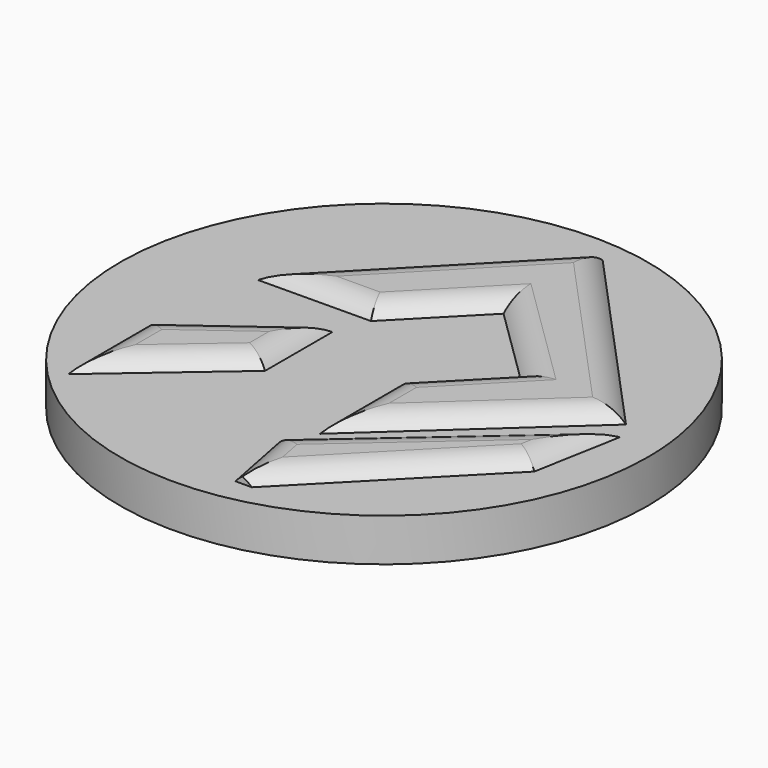
from build123d import *

# Parameters (mm, degrees)
F1_R         = 43.0886477689
F2_DEPTH     = 7
F3_DEPTH     = 9
F4_T1_DEPTH  = 65.4537906692
F4_T3_DEPTH  = 64.2896699852
F4_T5_DEPTH  = 38.3423168452
F4_T7_DEPTH  = 27.0257675551
F4_T9_DEPTH  = 18.685309
F4_T11_DEPTH = 25.5512004517
F4_T13_DEPTH = 59.0901082548
F4_T15_DEPTH = 43.6259466426
F4_T17_DEPTH = 36.1199672148
F4_T19_DEPTH = 45.1090392988
F4_T21_DEPTH = 31.581321794
F4_T23_DEPTH = 56.2861348222
F4_T25_DEPTH = 34.5042209979
F4_T27_DEPTH = 63.7210704382
F4_T32_DEPTH = 36.3207046716
F4_T37_DEPTH = 33.7416105717
F4_T43_DEPTH = 37.0257675551
F4_T47_DEPTH = 28.685309
F4_T54_DEPTH = 28.685309
F4_T58_DEPTH = 35.5512004517


# Not quite as in the source:
# - a fillet or chamfer that OpenCascade refuses, or shapes differently, is made with other operations: its cross-section is extruded or revolved along the edge and cut away or added


with BuildPart() as f2:
    # F1 (on Top) → F2 (new body)
    with BuildSketch(Plane.XY):
        with Locations((0, 9.9098170176)):
            Circle(F1_R)
    extrude(amount=F2_DEPTH)

    # F0 (on Top) → F3 (join)
    with BuildSketch(Plane.XY):
        Polygon((4.6245767735, 48.7562939525), (-26.2940470129, 17.0448832214), (-7.9522941785, 17.1887241356), (3.9733163334, 29.3401263082), (17.3091441393, 16.252098605), (6.4163865013, 5.1531046629), (6.4163865013, -11.1676000087), (35.278942436, 15.1950521395), align=None)
        Polygon((-9.9098188803, 11.7596480995), (-28.9366655052, -2.2462243214), (-28.9366655052, -18.3661915362), (-9.9098188803, -1.9819624722), align=None)
        Polygon((6.2101469375, -28.1438771635), (8.8527640328, -28.1438771635), (34.2691988262, -2.2462243214), (36.864515394, 12.0239108801), (3.9733163334, -16.7806204408), align=None)
    extrude(amount=F3_DEPTH)

    # F4: fillet of radius 5 on 17 edges, made by hand

    # F4_s2 → F4_t1 (cut)
    with BuildSketch(Plane(origin=(15.2233690689, -16.6669627471, 0), x_dir=(0, 0, 1), z_dir=(-0.6744072433, 0.7383595806, 0))):
        with BuildLine():
            ThreePointArc((7, 36.2961983644), (8.472135955, 34.5322663419), (9, 32.2961983644))
            Line((9, 32.2961983644), (9, 36.2961983644))
            Line((9, 36.2961983644), (7, 36.2961983644))
        make_face()
    extrude(amount=F4_T1_DEPTH, mode=Mode.SUBTRACT)

    # F4_s4 → F4_t3 (cut)
    with BuildSketch(Plane(origin=(33.6050957981, 34.4667667899, 0), x_dir=(0, 0, 1), z_dir=(-0.6981001167, -0.7160001585, 0))):
        with BuildLine():
            ThreePointArc((7, 30.7255767963), (8.472135955, 28.9616447738), (9, 26.7255767963))
            Line((9, 26.7255767963), (9, 30.7255767963))
            Line((9, 30.7255767963), (7, 30.7255767963))
        make_face()
    extrude(amount=F4_T3_DEPTH, mode=Mode.SUBTRACT)

    # F4_s6 → F4_t5 (cut)
    with BuildSketch(Plane(origin=(-36.1584602101, -0.2835642821, 0), x_dir=(0, 0, 1), z_dir=(0.9999692508, 0.0078420254, 0))):
        with BuildLine():
            ThreePointArc((7, -17.2505576897), (8.472135955, -19.0144897122), (9, -21.2505576897))
            Line((9, -21.2505576897), (9, -17.2505576897))
            Line((9, -17.2505576897), (7, -17.2505576897))
        make_face()
    extrude(amount=F4_T5_DEPTH, mode=Mode.SUBTRACT)

    # F4_s8 → F4_t7 (cut)
    with BuildSketch(Plane(origin=(-2.3131754341, -2.3569715754, 0), x_dir=(0, 0, 1), z_dir=(0.7004448095, 0.7137065705, 0))):
        with BuildLine():
            ThreePointArc((7, -17.7153572089), (8.472135955, -19.4792892314), (9, -21.7153572089))
            Line((9, -21.7153572089), (9, -17.7153572089))
            Line((9, -17.7153572089), (7, -17.7153572089))
        make_face()
    extrude(amount=F4_T7_DEPTH, mode=Mode.SUBTRACT)

    # F4_s10 → F4_t9 (cut)
    with BuildSketch(Plane(origin=(-12.6435668395, 12.4086300056, 0), x_dir=(0, 0, 1), z_dir=(0.7137065705, -0.7004448095, 0))):
        with BuildLine():
            ThreePointArc((7, -23.7233297289), (8.472135955, -25.4872617514), (9, -27.7233297289))
            Line((9, -27.7233297289), (9, -23.7233297289))
            Line((9, -23.7233297289), (7, -23.7233297289))
        make_face()
    extrude(amount=F4_T9_DEPTH, mode=Mode.SUBTRACT)

    # F4_s12 → F4_t11 (cut)
    with BuildSketch(Plane(origin=(16.6168831729, 16.9314963026, 0), x_dir=(0, 0, 1), z_dir=(-0.7004448095, -0.7137065705, 0))):
        with BuildLine():
            ThreePointArc((7, -0.9699517911), (8.472135955, -2.7338838136), (9, -4.9699517911))
            Line((9, -4.9699517911), (9, -0.9699517911))
            Line((9, -0.9699517911), (7, -0.9699517911))
        make_face()
    extrude(amount=F4_T11_DEPTH, mode=Mode.SUBTRACT)

    # F4_s14 → F4_t13 (cut)
    with BuildSketch(Plane(origin=(-9.4465059402, -8.6283055001, 0), x_dir=(0, 0, 1), z_dir=(0.7383595806, 0.6744072433, 0))):
        with BuildLine():
            ThreePointArc((7, 12.5729619904), (8.472135955, 10.8090299679), (9, 8.5729619904))
            Line((9, 8.5729619904), (9, 12.5729619904))
            Line((9, 12.5729619904), (7, 12.5729619904))
        make_face()
    extrude(amount=F4_T13_DEPTH, mode=Mode.SUBTRACT)

    # F4_s16 → F4_t15 (cut)
    with BuildSketch(Plane(origin=(7.2404468524, 5.3297730772, 0), x_dir=(0, 0, 1), z_dir=(-0.8053368998, -0.5928174068, 0))):
        with BuildLine():
            ThreePointArc((7, 15.3451916737), (8.472135955, 13.5812596512), (9, 11.3451916737))
            Line((9, 11.3451916737), (9, 15.3451916737))
            Line((9, 15.3451916737), (7, 15.3451916737))
        make_face()
    extrude(amount=F4_T15_DEPTH, mode=Mode.SUBTRACT)

    # F4_s18 → F4_t17 (cut)
    with BuildSketch(Plane.XZ.offset(-7.7537756786)):
        with BuildLine():
            ThreePointArc((-28.9366655052, 7), (-27.1727334827, 8.472135955), (-24.9366655052, 9))
            Line((-24.9366655052, 9), (-28.9366655052, 9))
            Line((-28.9366655052, 9), (-28.9366655052, 7))
        make_face()
    extrude(amount=F4_T17_DEPTH, mode=Mode.SUBTRACT)

    # F4_s20 → F4_t19 (cut)
    with BuildSketch(Plane(origin=(-33.2748914759, -28.6533788161, 0), x_dir=(0, 0, 1), z_dir=(0.7577688018, 0.652523136, 0))):
        with BuildLine():
            ThreePointArc((7, -4.9645167646), (8.472135955, -6.7284487871), (9, -8.9645167646))
            Line((9, -8.9645167646), (9, -4.9645167646))
            Line((9, -4.9645167646), (7, -4.9645167646))
        make_face()
    extrude(amount=F4_T19_DEPTH, mode=Mode.SUBTRACT)

    # F4_s22 → F4_t21 (cut)
    with BuildSketch(Plane(origin=(1.3968105752, -7.0958959209, 0), x_dir=(0, 0, 1), z_dir=(0.1931412186, -0.9811709686, 0))):
        with BuildLine():
            ThreePointArc((7, -0.657473155), (8.472135955, -2.4214051775), (9, -4.657473155))
            Line((9, -4.657473155), (9, -0.657473155))
            Line((9, -0.657473155), (7, -0.657473155))
        make_face()
    extrude(amount=F4_T21_DEPTH, mode=Mode.SUBTRACT)

    # F4_s24 → F4_t23 (cut)
    with BuildSketch(Plane(origin=(-16.7305427457, -17.047307831, 0), x_dir=(0, 0, 1), z_dir=(0.7004448095, 0.7137065705, 0))):
        with BuildLine():
            ThreePointArc((7, 26.0315085363), (8.472135955, 24.2675765138), (9, 22.0315085363))
            Line((9, 22.0315085363), (9, 26.0315085363))
            Line((9, 26.0315085363), (7, 26.0315085363))
        make_face()
    extrude(amount=F4_T23_DEPTH, mode=Mode.SUBTRACT)

    # F4_s26 → F4_t25 (cut)
    with BuildSketch(Plane(origin=(-1.0875692561, -5.9799103194, 0), x_dir=(0, 0, 1), z_dir=(0.1789352609, 0.9838608501, 0))):
        with BuildLine():
            ThreePointArc((7, 34.1180518253), (8.472135955, 32.3541198028), (9, 30.1180518253))
            Line((9, 30.1180518253), (9, 34.1180518253))
            Line((9, 34.1180518253), (7, 34.1180518253))
        make_face()
    extrude(amount=F4_T25_DEPTH, mode=Mode.SUBTRACT)

    # F4_s28 → F4_t27 (cut)
    with BuildSketch(Plane(origin=(34.3458542038, 30.0784483818, 0), x_dir=(0, 0, 1), z_dir=(-0.7522962894, -0.6588249334, 0))):
        with BuildLine():
            ThreePointArc((7, -15.2417183608), (8.472135955, -17.0056503833), (9, -19.2417183608))
            Line((9, -19.2417183608), (9, -15.2417183608))
            Line((9, -15.2417183608), (7, -15.2417183608))
        make_face()
    extrude(amount=F4_T27_DEPTH, mode=Mode.SUBTRACT)


with BuildPart() as f4_tool30:
    # F4_s31 → F4_t32 (new body)
    with BuildSketch(Plane.XZ.offset(-15.1531046629)):
        with BuildLine():
            ThreePointArc((6.4163865013, 7), (8.1803185238, 8.472135955), (10.4163865013, 9))
            Line((10.4163865013, 9), (6.4163865013, 9))
            Line((6.4163865013, 9), (6.4163865013, 7))
        make_face()
    extrude(amount=F4_T32_DEPTH)

    split(bisect_by=Plane(origin=(8.479296636, -9.2833669415, 0), x_dir=(0, 0, 1), z_dir=(-0.6744072433, 0.7383595806, 0)), keep=Keep.TOP)


with BuildPart() as f2_1:
    add(f2.part)

    # F4_t29: cut F4_tool30
    add(f4_tool30.part, mode=Mode.SUBTRACT)


with BuildPart() as f4_tool35:
    # F4_s36 → F4_t37 (new body)
    with BuildSketch(Plane.XZ.offset(11.9819624722)):
        with BuildLine():
            ThreePointArc((-9.9098188803, 7), (-11.6737509028, 8.472135955), (-13.9098188803, 9))
            Line((-13.9098188803, 9), (-9.9098188803, 9))
            Line((-9.9098188803, 9), (-9.9098188803, 7))
        make_face()
    extrude(amount=-F4_T37_DEPTH)

    split(bisect_by=Plane(origin=(-0.1352793112, 17.2500272496, 0), x_dir=(0, 0, 1), z_dir=(0.0078420254, -0.9999692508, 0)), keep=Keep.TOP)


with BuildPart() as f2_2:
    add(f2_1.part)

    # F4_t34: cut F4_tool35
    add(f4_tool35.part, mode=Mode.SUBTRACT)


with BuildPart() as f4_tool41:
    # F4_s42 → F4_t43 (new body)
    with BuildSketch(Plane(origin=(-2.3131754341, -2.3569715754, 0), x_dir=(0, 0, 1), z_dir=(0.7004448095, 0.7137065705, 0))):
        with BuildLine():
            ThreePointArc((7, -17.7153572089), (8.472135955, -19.4792892314), (9, -21.7153572089))
            Line((9, -21.7153572089), (9, -17.7153572089))
            Line((9, -17.7153572089), (7, -17.7153572089))
        make_face()
    extrude(amount=F4_T43_DEPTH)

    split(bisect_by=Plane(origin=(16.6168831729, 16.9314963026, 0), x_dir=(0, 0, 1), z_dir=(0.7004448095, 0.7137065705, 0)), keep=Keep.TOP)


with BuildPart() as f4_tool45:
    # F4_s46 → F4_t47 (new body)
    with BuildSketch(Plane(origin=(-19.7806325449, 19.4130781007, 0), x_dir=(0, 0, 1), z_dir=(0.7137065705, -0.7004448095, 0))):
        with BuildLine():
            ThreePointArc((7, -23.7233297289), (8.472135955, -25.4872617514), (9, -27.7233297289))
            Line((9, -27.7233297289), (9, -23.7233297289))
            Line((9, -23.7233297289), (7, -23.7233297289))
        make_face()
    extrude(amount=F4_T47_DEPTH)

    split(bisect_by=Plane(origin=(-12.6435668395, 12.4086300056, 0), x_dir=(0, 0, 1), z_dir=(-0.7137065705, 0.7004448095, 0)), keep=Keep.TOP)


with BuildPart() as f4_tool41_1:
    add(f4_tool41.part)

    # F4_t49: intersect F4_tool45
    add(f4_tool45.part, mode=Mode.INTERSECT)


with BuildPart() as f2_3:
    add(f2_2.part)

    # F4_t39: cut F4_tool41
    add(f4_tool41_1.part, mode=Mode.SUBTRACT)


with BuildPart() as f4_tool52:
    # F4_s53 → F4_t54 (new body)
    with BuildSketch(Plane(origin=(-12.6435668395, 12.4086300056, 0), x_dir=(0, 0, 1), z_dir=(0.7137065705, -0.7004448095, 0))):
        with BuildLine():
            ThreePointArc((7, -23.7233297289), (8.472135955, -25.4872617514), (9, -27.7233297289))
            Line((9, -27.7233297289), (9, -23.7233297289))
            Line((9, -23.7233297289), (7, -23.7233297289))
        make_face()
    extrude(amount=F4_T54_DEPTH)

    split(bisect_by=Plane(origin=(0.6922609664, -0.6793976976, 0), x_dir=(0, 0, 1), z_dir=(0.7137065705, -0.7004448095, 0)), keep=Keep.TOP)


with BuildPart() as f4_tool56:
    # F4_s57 → F4_t58 (new body)
    with BuildSketch(Plane(origin=(23.621331268, 24.068562008, 0), x_dir=(0, 0, 1), z_dir=(-0.7004448095, -0.7137065705, 0))):
        with BuildLine():
            ThreePointArc((7, -0.9699517911), (8.472135955, -2.7338838136), (9, -4.9699517911))
            Line((9, -4.9699517911), (9, -0.9699517911))
            Line((9, -0.9699517911), (7, -0.9699517911))
        make_face()
    extrude(amount=F4_T58_DEPTH)

    split(bisect_by=Plane(origin=(16.6168831729, 16.9314963026, 0), x_dir=(0, 0, 1), z_dir=(0.7004448095, 0.7137065705, 0)), keep=Keep.TOP)


with BuildPart() as f4_tool52_1:
    add(f4_tool52.part)

    # F4_t60: intersect F4_tool56
    add(f4_tool56.part, mode=Mode.INTERSECT)


with BuildPart() as f2_4:
    add(f2_3.part)

    # F4_t50: cut F4_tool52
    add(f4_tool52_1.part, mode=Mode.SUBTRACT)


solid = f2_4.part
